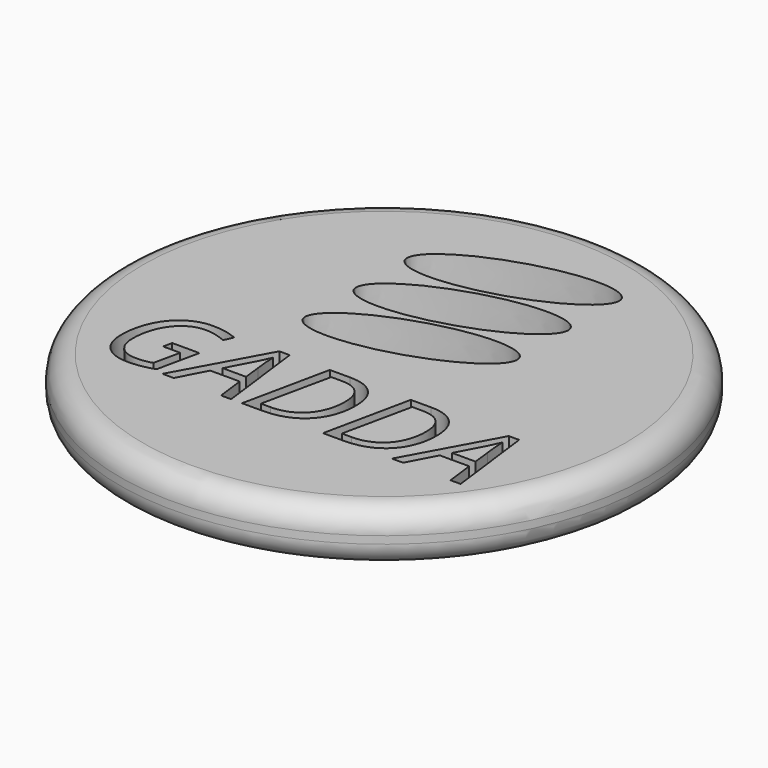
from build123d import *

# Parameters (mm, degrees)
F1_R         = 11.625
F2_DEPTH     = 2.33
F3_R         = 1
F4_TEXT_SIZE = 5.3548916993
F6_DEPTH     = 2.33
F7_DEPTH     = 2.33


# Not quite as in the source:
# - Text() gives the source's letters only with a copy of the font that has no kerning and outlines rounded to 1/6400 em; it was checked with that copy


with BuildPart() as f2:
    # F1 (on Top) → F2 (new body)
    with BuildSketch(Plane.XY):
        Circle(F1_R)
    extrude(amount=F2_DEPTH)

    # F3
    f3_edges = [f2.edges().sort_by_distance(p)[0] for p in [
        (-11.625, 0, 0),
        (-11.625, 0, 2.33),
    ]]
    fillet(f3_edges, radius=F3_R)

    # F4 (on Top) → F6 (cut, through all)
    with BuildSketch(Plane.XY):
        with Locations((-8.343255613, -5.9203777928)):
            Text('GADDA', F4_TEXT_SIZE, font='Open Sans', font_style=FontStyle.ITALIC, text_align=(TextAlign.LEFT, TextAlign.BOTTOM))
    extrude(amount=F6_DEPTH, mode=Mode.SUBTRACT)

    # F5 (on face) → F7 (cut, through all)
    with BuildSketch(Plane.XY.offset(2.33)):
        with BuildLine():
            add(Edge.make_bspline(
                [(3.8310968506, 8.2583576682), (3.2085947512, 10.3319996663), (-2.226799475, 7.5700502449), (-7.6621937011, 4.8081008235), (-1.6042973756, 5.4964082468), (4.45359895, 6.1847156701), (3.8310968506, 8.2583576682)],
                knots=[0, 0, 0, 2.0943951024, 2.0943951024, 4.1887902048, 4.1887902048, 6.2831853072, 6.2831853072, 6.2831853072], degree=2, weights=[1, 0.5, 1, 0.5, 1, 0.5, 1]))
        make_face()
        with BuildLine():
            add(Edge.make_bspline(
                [(3.8310968506, 5.4500856149), (3.2085947512, 7.523727613), (-2.226799475, 4.7617781916), (-7.6621937011, 1.9998287702), (-1.6042973756, 2.6881361935), (4.45359895, 3.3764436168), (3.8310968506, 5.4500856149)],
                knots=[0, 0, 0, 2.0943951024, 2.0943951024, 4.1887902048, 4.1887902048, 6.2831853072, 6.2831853072, 6.2831853072], degree=2, weights=[1, 0.5, 1, 0.5, 1, 0.5, 1]))
        make_face()
        with BuildLine():
            add(Edge.make_bspline(
                [(3.8310968506, 2.6418135616), (3.2085947512, 4.7154555597), (-2.226799475, 1.9535061383), (-7.6621937011, -0.8084432831), (-1.6042973756, -0.1201358598), (4.45359895, 0.5681715635), (3.8310968506, 2.6418135616)],
                knots=[0, 0, 0, 2.0943951024, 2.0943951024, 4.1887902048, 4.1887902048, 6.2831853072, 6.2831853072, 6.2831853072], degree=2, weights=[1, 0.5, 1, 0.5, 1, 0.5, 1]))
        make_face()
    extrude(amount=-F7_DEPTH, mode=Mode.SUBTRACT)


solid = f2.part
